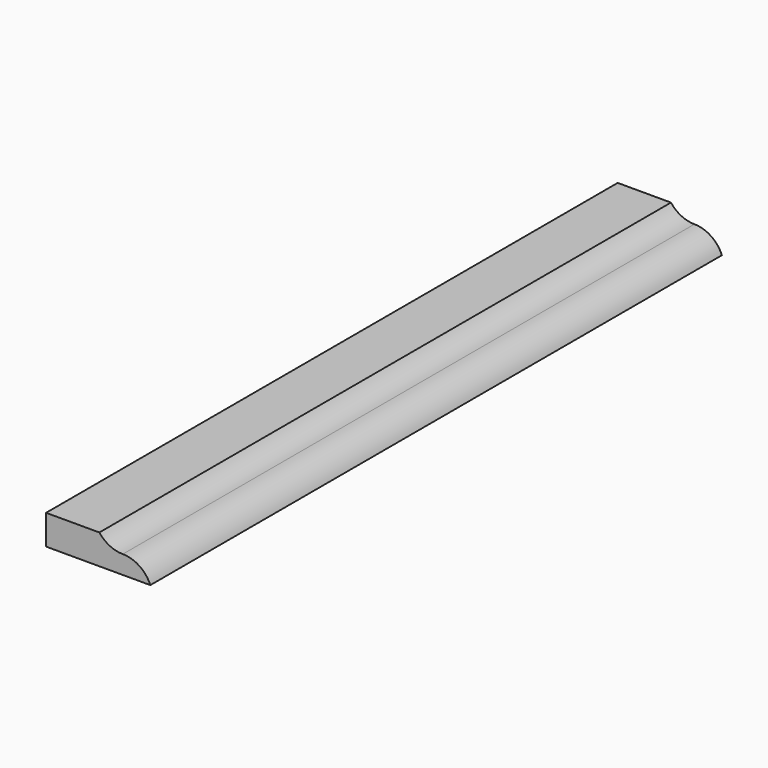
from build123d import *

# Parameters (mm, degrees)
F1_DEPTH = 152.4


# Not quite as in the source:
# - ends of sketch curves that miss each other by under 0.0002 mm in the source are joined


with BuildPart() as f1:
    # F0 (on Front) → F1 (new body)
    with BuildSketch(Plane.XZ):
        with BuildLine():
            Line((0.247523, 3.176651), (-11.1182404, 3.176651))
            Line((-11.1182404, 3.176651), (-11.1182404, -3.1766256))
            Line((-11.1182404, -3.1766256), (11.1182404, -3.1766256))
            ThreePointArc((11.1182404, -3.1766256), (8.7779959458, -0.3307242374), (5.2517548, 0.7376922))
            ThreePointArc((5.2517548, 0.7376922), (2.4682848878, 1.3798901975), (0.247523, 3.176651))
        make_face()
    extrude(amount=F1_DEPTH)


solid = f1.part
